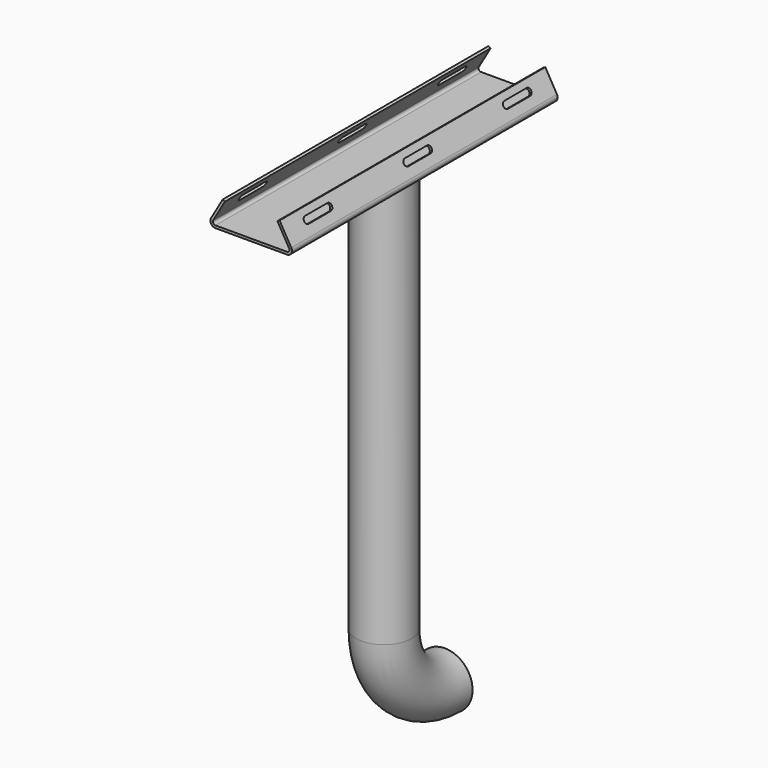
from build123d import *

# Parameters (mm, degrees)
F1_DEPTH = 304.8
F5_R     = 25.4
F5_R_2   = 23.114
F8_DEPTH = 2.286


# Not quite as in the source:
# - a pattern or mirror of a feature is missing from the dataset's text; its kind, count and spacing are read off the source's solid


with BuildPart() as f1:
    # F0 (on Front) → F1 (new body)
    with BuildSketch(Plane.XZ):
        with BuildLine():
            ThreePointArc((-36.8149627644, 6.858), (-36.8149627644, 2.286), (-32.8554946183, 0))
            Line((-32.8554946183, 0), (32.8554946183, 0))
            ThreePointArc((32.8554946183, 0), (36.8149627644, 2.286), (36.8149627644, 6.858))
            Line((36.8149627644, 6.858), (26.1097340731, 25.4))
            Line((26.1097340731, 25.4), (24.13, 24.257))
            Line((24.13, 24.257), (34.8352286913, 5.715))
            ThreePointArc((34.8352286913, 5.715), (34.8352286913, 3.429), (32.8554946183, 2.286))
            Line((32.8554946183, 2.286), (-32.8554946183, 2.286))
            ThreePointArc((-32.8554946183, 2.286), (-34.8352286913, 3.429), (-34.8352286913, 5.715))
            Line((-34.8352286913, 5.715), (-24.13, 24.257))
            Line((-24.13, 24.257), (-26.1097340731, 25.4))
            Line((-26.1097340731, 25.4), (-36.8149627644, 6.858))
        make_face()
    extrude(amount=F1_DEPTH)

    # F6: sweep along a path in F3
    with BuildLine(Plane.YZ) as f6_path:
        Line((-152.4, 0), (-152.4, -374.65))
        ThreePointArc((-152.4, -374.65), (-131.9414086659, -424.0414086659), (-82.55, -444.5))
    # F5 (on plane+point) → F6 (sweep)
    with BuildSketch(Plane.XZ.offset(82.55)):
        with Locations((0, -444.5)):
            Circle(F5_R)
        with Locations((0, -444.5)):
            Circle(F5_R_2, mode=Mode.SUBTRACT)
    sweep(path=f6_path.line)

    # F7 (on face) → F8 (cut, through all)
    with BuildSketch(Plane(origin=(30.5808231829, 0, 17.6558464967), x_dir=(0, 1, 0), z_dir=(0.8660254038, 0, 0.5))):
        with BuildLine():
            Line((-254, 2.5921782196), (-279.4, 2.5921782196))
            ThreePointArc((-279.4, 2.5921782196), (-282.575, -0.5828217804), (-279.4, -3.7578217804))
            Line((-279.4, -3.7578217804), (-254, -3.7578217804))
            ThreePointArc((-254, -3.7578217804), (-250.825, -0.5828217804), (-254, 2.5921782196))
        make_face()
        with BuildLine():
            Line((-139.7, 2.5921782196), (-165.1, 2.5921782196))
            ThreePointArc((-165.1, 2.5921782196), (-168.275, -0.5828217804), (-165.1, -3.7578217804))
            Line((-165.1, -3.7578217804), (-139.7, -3.7578217804))
            ThreePointArc((-139.7, -3.7578217804), (-136.525, -0.5828217804), (-139.7, 2.5921782196))
        make_face()
        with BuildLine():
            ThreePointArc((-25.4, -3.7578217804), (-22.225, -0.5828217804), (-25.4, 2.5921782196))
            Line((-25.4, 2.5921782196), (-50.8, 2.5921782196))
            ThreePointArc((-50.8, 2.5921782196), (-53.975, -0.5828217804), (-50.8, -3.7578217804))
            Line((-50.8, -3.7578217804), (-25.4, -3.7578217804))
        make_face()
    f8 = extrude(amount=-F8_DEPTH, mode=Mode.SUBTRACT)

    # F8_copies: F8 across plane
    add(f8.mirror(Plane(origin=(0, 0, 0), x_dir=(0, 0, -1), z_dir=(-1, 0, 0))), mode=Mode.SUBTRACT)


solid = f1.part
